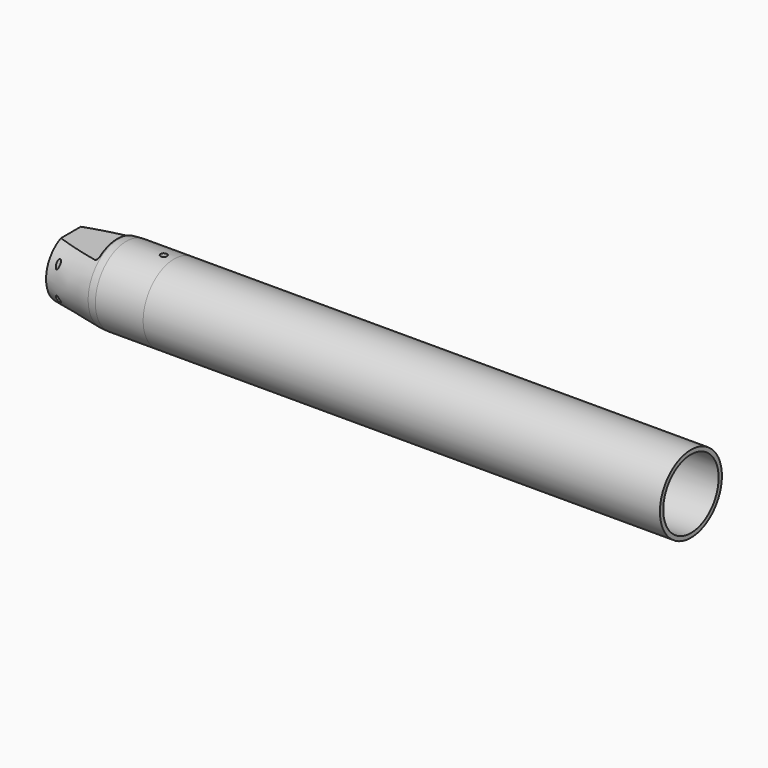
from build123d import *

# Parameters (mm, degrees)
F6_D          = 8.334375
F7_R          = 0.79375
F8_DEPTH      = 9.526
F8_DEPTH_BACK = 9.526
F9_R          = 12.7
F10_R         = 4.1402
F10_R_2       = 3.175
F11_DEPTH     = 12.7
F13_DEPTH     = 11.43
F14_R         = 0.762
F15_R         = 0.508
F16_DEPTH     = 16.5110001


# Not quite as in the source:
# - a length typed as a fraction of an inch, garbled in the dataset ("3 / 203.2 mm" for 3/8 in), is restored


with BuildPart() as f2:
    # F0 (on Top) → F2 (revolve)
    with BuildSketch(Plane.XY):
        Polygon((127, 9.525), (0, 9.525), (0, 8.509), (12.7, 8.509), (12.7, 8.382), (114.3, 8.382), (114.3, 8.509), (127, 8.509), align=None)
    revolve(axis=Axis((12.7, 0, 0), (1, 0, 0)))


with BuildPart() as f4:
    # F3 (on Top) → F4 (revolve)
    with BuildSketch(Plane.XY):
        with BuildLine():
            Line((-25.4, 7.62), (-25.4, 0))
            Line((-25.4, 0), (-12.7, 0))
            Line((-12.7, 0), (-12.7, 4.445))
            ThreePointArc((-12.7, 4.445), (-12.2536307345, 5.5226307345), (-11.176, 5.969))
            Line((-11.176, 5.969), (8.89, 5.969))
            Line((8.89, 5.969), (8.89, 8.509))
            Line((8.89, 8.509), (0, 8.509))
            Line((0, 8.509), (0, 9.525))
            Line((0, 9.525), (-12.7, 9.525))
            Line((-12.7, 9.525), (-25.4, 7.62))
        make_face()
    revolve(axis=Axis((12.7, 0, 0), (1, 0, 0)))

    # F6 (through all)
    with Locations(Plane(origin=(-25.4, 0, 0), x_dir=(0, -1, 0), z_dir=(-1, 0, 0))):
        with Locations((0, 0)):
            Hole(F6_D / 2)

    # F7 (on Top) → F8 (cut, two sides)
    with BuildSketch(Plane.XY) as f8_sk:
        with Locations((-2.54, 0)):
            Circle(F7_R)
    extrude(amount=-F8_DEPTH, mode=Mode.SUBTRACT)
    extrude(f8_sk.sketch, amount=F8_DEPTH_BACK, mode=Mode.SUBTRACT)

    # F9
    f9_edges = [f4.edges().sort_by_distance(p)[0] for p in [
        (-12.7, -9.525, 0),
    ]]
    fillet(f9_edges, radius=F9_R)

    # F12 (on face) → F13 (cut)
    with BuildSketch(Plane(origin=(-25.4, 0, 0), x_dir=(0, -1, 0), z_dir=(-1, 0, 0))):
        with BuildLine():
            ThreePointArc((6.4757547823, 6.985), (0, 9.525), (-6.4757547823, 6.985))
            Line((-6.4757547823, 6.985), (6.4757547823, 6.985))
        make_face()
        with BuildLine():
            Line((6.4757547823, -6.985), (-6.4757547823, -6.985))
            ThreePointArc((-6.4757547823, -6.985), (0, -9.525), (6.4757547823, -6.985))
        make_face()
    extrude(amount=-F13_DEPTH, mode=Mode.SUBTRACT)

    # F14
    f14_edges = [f4.edges().sort_by_distance(p)[0] for p in [
        (-13.97, 0, 6.985),
        (-13.97, 0, -6.985),
    ]]
    fillet(f14_edges, radius=F14_R)

    # F15 (on face) → F16 (cut, through all)
    with BuildSketch(Plane.XY.offset(6.985)):
        with Locations((-22.86, 6.985)):
            Circle(F15_R)
        with Locations((-22.86, -6.985)):
            Circle(F15_R)
    extrude(amount=-F16_DEPTH, mode=Mode.SUBTRACT)


with BuildPart() as f11:
    # F10 (on face) → F11 (new body)
    with BuildSketch(Plane(origin=(-25.4, 0, 0), x_dir=(0, -1, 0), z_dir=(-1, 0, 0))):
        Circle(F10_R)
        Circle(F10_R_2, mode=Mode.SUBTRACT)
    extrude(amount=-F11_DEPTH)


solid = Compound([f2.part, f4.part, f11.part])
